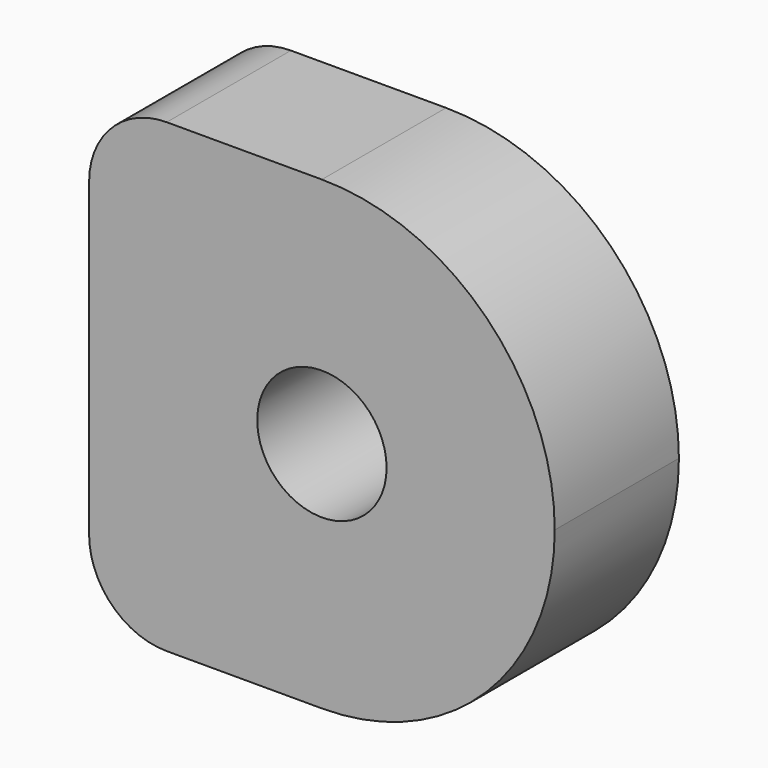
from build123d import *

# Parameters (mm, degrees)
F0_R     = 2.5
F1_DEPTH = 6
F2_R     = 3


with BuildPart() as f1:
    # F0 (on Front) → F1 (new body)
    with BuildSketch(Plane.XZ):
        with BuildLine():
            Line((0, 9), (0, 0))
            Line((0, 0), (9, 0))
            ThreePointArc((9, 0), (2.6360389693, 2.6360389693), (0, 9))
        make_face()
        with BuildLine():
            ThreePointArc((0, 9), (2.6360389693, 2.6360389693), (9, 0))
            ThreePointArc((9, 0), (15.3639610307, 2.6360389693), (18, 9))
            ThreePointArc((18, 9), (15.3639610307, 15.3639610307), (9, 18))
            ThreePointArc((9, 18), (2.6360389693, 15.3639610307), (0, 9))
        make_face()
        with Locations((9, 9)):
            Circle(F0_R, mode=Mode.SUBTRACT)
        with BuildLine():
            Line((0, 18), (0, 9))
            ThreePointArc((0, 9), (2.6360389693, 15.3639610307), (9, 18))
            Line((9, 18), (0, 18))
        make_face()
    extrude(amount=F1_DEPTH)

    # F2
    f2_edges = [f1.edges().sort_by_distance(p)[0] for p in [
        (0, -3, 18),
        (0, -3, 0),
    ]]
    fillet(f2_edges, radius=F2_R)


solid = f1.part
